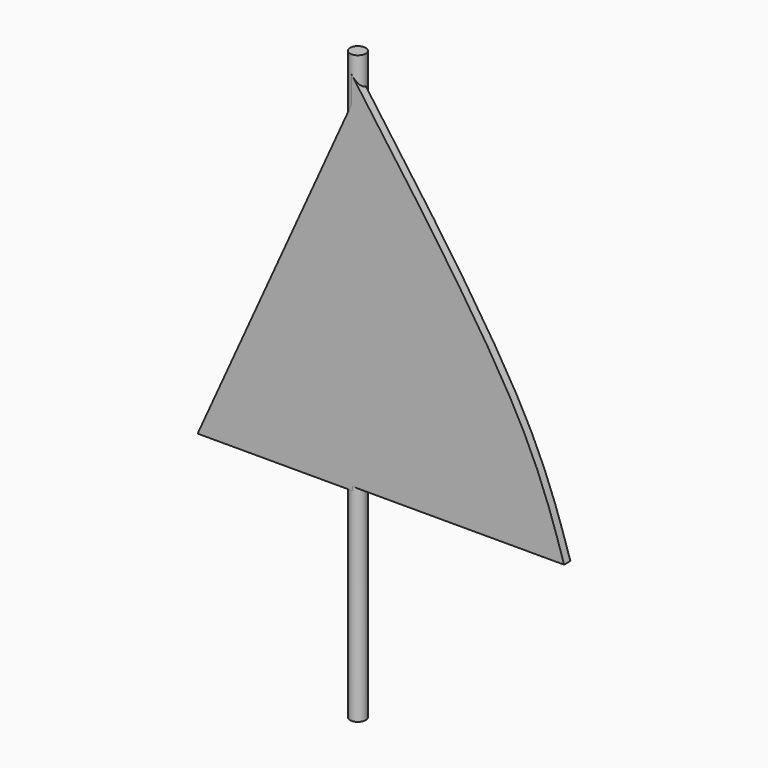
from build123d import *

# Parameters (mm, degrees)
F1_W     = 2
F1_H     = 150
F5_DEPTH = 2
F7_DEPTH = 2


# Not quite as in the source:
# - the program builds the solid bodies; features that only make, move or delete a surface that nothing else refers to are left out


with BuildPart() as f4:
    # F1 (on Front) → F4 (revolve)
    with BuildSketch(Plane.XZ):
        with Locations((-1, -7.0591911674)):
            Rectangle(F1_W, F1_H)
    revolve(axis=Axis((0, 0, 16.0941202193), (0, 0, -1)))

    # F0 (on Front) → F5 (join)
    with BuildSketch(Plane.XZ):
        with BuildLine():
            Line((0, 63.3778050542), (0, -29.2516257614))
            Line((0, -29.2516257614), (54.3039664626, -29.2516257614))
            add(Edge.make_bspline(
                [(0, 63.3778050542), (16.6847622445, 40.4423802167), (44.0846316514, 2.7776154372), (51.4310467474, -20.2473764435), (54.3039664626, -29.2516257614)],
                knots=[0, 0, 0, 0, 0.6089358309, 1, 1, 1, 1], degree=3))
        make_face()
    extrude(amount=F5_DEPTH)

    # F2 (on Front) → F7 (join)
    with BuildSketch(Plane.XZ):
        Polygon((0.1667886972, -30.2148442715), (0, 56.7073263228), (-39.3750006333, -30.2148442715), align=None)
    extrude(amount=F7_DEPTH)


solid = f4.part
